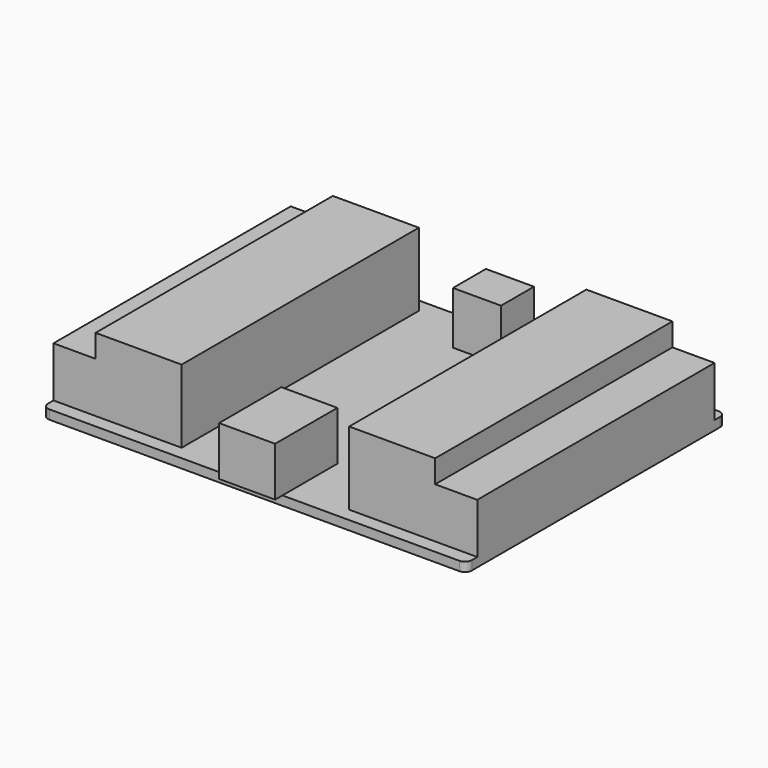
from build123d import *

# Parameters (mm, degrees)
F0_W      = 92.61
F0_H      = 70.8
F1_DEPTH  = 2
F2_W      = 28
F2_H      = 64.8
F3_DEPTH  = 16
F4_W      = 9.2
F4_H      = 64.8
F5_DEPTH  = 5
F7_W      = 12.25
F7_H      = 15
F8_DEPTH  = 10.75
F9_R      = 1.5
F10_W     = 12.25
F10_H     = 10.75
F11_DEPTH = 2
F12_W     = 10.5
F12_H     = 9
F13_DEPTH = 11.5


# Not quite as in the source:
# - a pattern or mirror of a feature is missing from the dataset's text; its kind, count and spacing are read off the source's solid


with BuildPart() as f1:
    # F0 (on Top) → F1 (new body)
    with BuildSketch(Plane.XY):
        with Locations((46.305, 35.4)):
            Rectangle(F0_W, F0_H)
    extrude(amount=F1_DEPTH)

    # F2 (on face) → F3 (join)
    with BuildSketch(Plane.XY.offset(2)):
        with Locations((78.61, 35.4)):
            Rectangle(F2_W, F2_H)
    f3 = extrude(amount=F3_DEPTH)

    # F3_copies: F3 across plane
    add(f3.mirror(Plane(origin=(46.305, 0, 0), x_dir=(0, 0, -1), z_dir=(-1, 0, 0))))

    # F4 (on face) → F5 (cut)
    with BuildSketch(Plane.XY.offset(18)):
        with Locations((88.01, 35.4)):
            Rectangle(F4_W, F4_H)
    f5 = extrude(amount=-F5_DEPTH, mode=Mode.SUBTRACT)

    # F5_copies: F5 across plane
    add(f5.mirror(Plane(origin=(46.305, 0, 0), x_dir=(0, 0, -1), z_dir=(-1, 0, 0))), mode=Mode.SUBTRACT)

    # F7 (on face) → F8 (join)
    with BuildSketch(Plane.XY.offset(2)):
        with Locations((46.305, 7.5)):
            Rectangle(F7_W, F7_H)
    extrude(amount=F8_DEPTH)

    # F9
    f9_edges = [f1.edges().sort_by_distance(p)[0] for p in [
        (92.61, 70.8, 1),
        (0, 70.8, 1),
        (0, 0, 1),
        (92.61, 0, 1),
    ]]
    fillet(f9_edges, radius=F9_R)

    # F10 (on face) → F11 (join)
    with BuildSketch(Plane.XZ):
        with Locations((46.305, 7.375)):
            Rectangle(F10_W, F10_H)
    extrude(amount=F11_DEPTH)

    # F12 (on face) → F13 (join)
    with BuildSketch(Plane.XY.offset(2)):
        with Locations((46.305, 65.3)):
            Rectangle(F12_W, F12_H)
    extrude(amount=F13_DEPTH)


solid = f1.part
